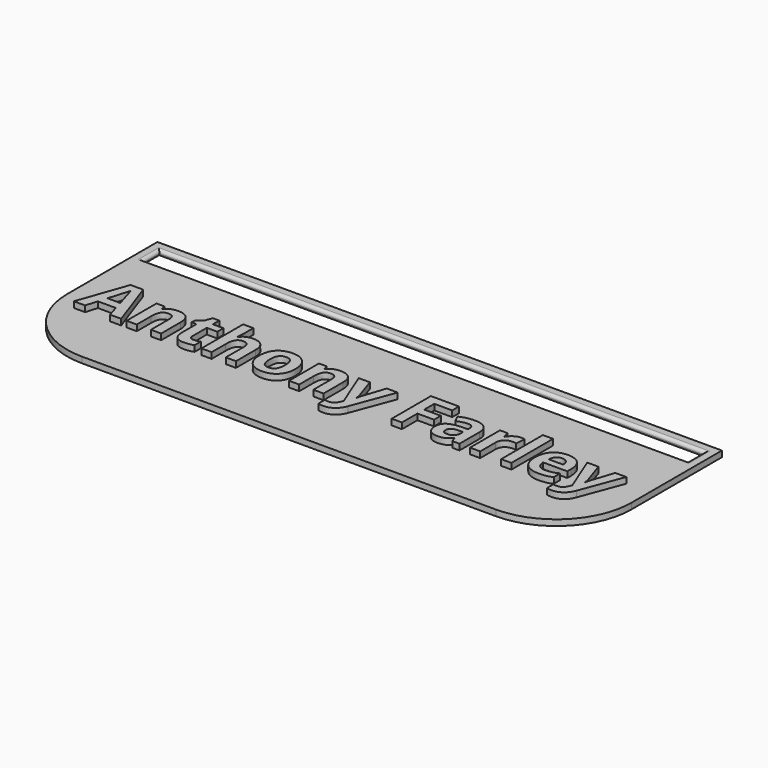
from build123d import *

# Parameters (mm, degrees)
F0_W         = 190.5
F0_H         = 63.5
F1_DEPTH     = 2
F2_W         = 183.896
F2_H         = 7.62
F3_DEPTH     = 25.4
F4_R         = 0.99999
F5_R         = 0.99999
F6_R         = 25.4
F7_TEXT_SIZE = 23.1500996867
F8_DEPTH     = 2


# Not quite as in the source:
# - a fillet or chamfer is up to 0.001 mm smaller than in the source, because OpenCascade refuses the exact size
# - Text() gives the source's letters only with a copy of the font that has no kerning and outlines rounded to 1/6400 em; it was checked with that copy


with BuildPart() as f1:
    # F0 (on Top) → F1 (new body)
    with BuildSketch(Plane.XY):
        with Locations((1.791532172, 31.75)):
            Rectangle(F0_W, F0_H)
    extrude(amount=F1_DEPTH)

    # F2 (on face) → F3 (cut)
    with BuildSketch(Plane.XY.offset(2)):
        with Locations((1.791532172, 56.388)):
            Rectangle(F2_W, F2_H)
    extrude(amount=-F3_DEPTH, mode=Mode.SUBTRACT)

    # F4 (radius 1 in the source; OpenCascade refuses exactly that, so slightly less here)
    f4_edges = [f1.edges().sort_by_distance(p)[0] for p in [
        (1.791532, 60.198, 2),
        (1.791532, 60.198, 0),
    ]]
    fillet(f4_edges, radius=F4_R)

    # F5 (radius 1 in the source; OpenCascade refuses exactly that, so slightly less here)
    f5_edges = [f1.edges().sort_by_distance(p)[0] for p in [
        (93.739532, 56.388, 0),
        (93.739532, 56.388, 2),
        (-90.156468, 56.388, 2),
        (-90.156468, 56.388, 0),
    ]]
    fillet(f5_edges, radius=F5_R)

    # F6
    f6_edges = [f1.edges().sort_by_distance(p)[0] for p in [
        (97.041532, 0, 1),
        (-93.458468, 0, 1),
    ]]
    fillet(f6_edges, radius=F6_R)

    # F7 (on face) → F8 (join)
    with BuildSketch(Plane.XY.offset(2)):
        with Locations((-87.108467828, 20.32)):
            Text('Anthony Farley', F7_TEXT_SIZE, font='Open Sans', font_style=FontStyle.BOLD, text_align=(TextAlign.LEFT, TextAlign.BOTTOM))
    extrude(amount=F8_DEPTH)


solid = f1.part
